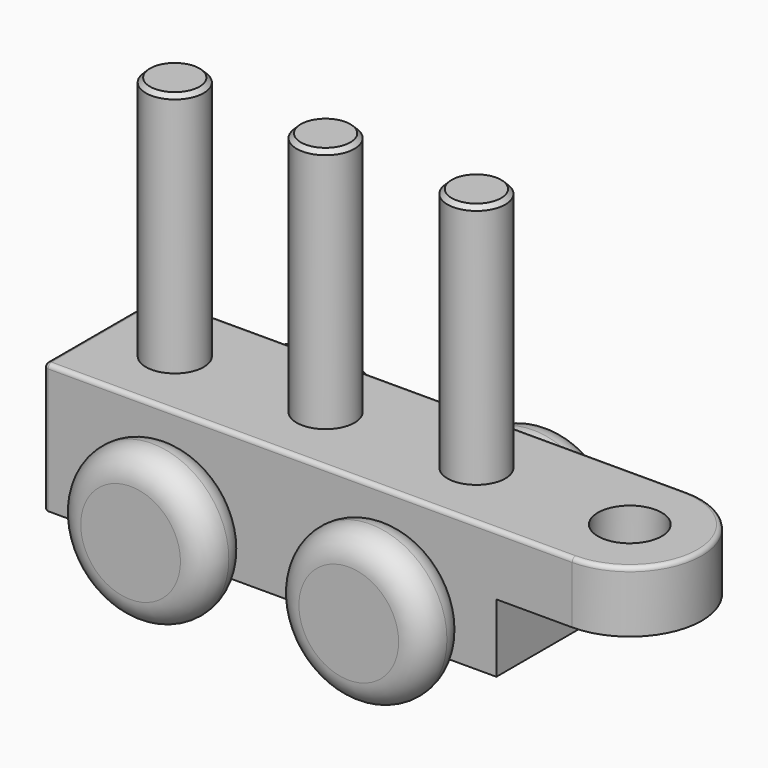
from build123d import *

# Parameters (mm, degrees)
F0_R           = 9.525
F1_DEPTH       = 38.608
F2_R           = 9.525
F3_DEPTH       = 20.32
F4_R           = 6.35
F5_DEPTH       = 42.926
F6_R           = 8.636
F7_DEPTH       = 73.152
F8_SIZE        = 1.27
F9_R           = 1.27
F10_R          = 6.35
F11_DEPTH      = 36.83
F12_R          = 22.86
F13_DEPTH      = 1.524
F13_DEPTH_BACK = 14.478
F12_R_2        = 6.35
F14_R          = 22.86
F14_R_2        = 6.35
F15_DEPTH      = 1.524
F15_DEPTH_BACK = 14.478
F16_R          = 8.00099
F16_2_R        = 8.00099
F16_3_R        = 8.00099
F16_4_R        = 8.00099


# Not quite as in the source:
# - a fillet or chamfer is up to 0.001 mm smaller than in the source, because OpenCascade refuses the exact size


with BuildPart() as f1:
    # F0 (on Top) → F1 (new body)
    with BuildSketch(Plane.XY):
        with BuildLine():
            Line((-21.463, 21.463), (-178.943, 21.463))
            Line((-178.943, 21.463), (-178.943, -21.463))
            Line((-178.943, -21.463), (-21.463, -21.463))
            ThreePointArc((-21.463, -21.463), (0, 0), (-21.463, 21.463))
        make_face()
        with Locations((-21.463, 0)):
            Circle(F0_R, mode=Mode.SUBTRACT)
    extrude(amount=F1_DEPTH)

    # F2 (on face) → F3 (cut)
    with BuildSketch(Plane(origin=(0, 0, 0), x_dir=(1, 0, 0), z_dir=(0, 0, -1))):
        with BuildLine():
            Line((-21.463, 21.463), (-44.069, 21.463))
            Line((-44.069, 21.463), (-44.069, -21.463))
            Line((-44.069, -21.463), (-21.463, -21.463))
            ThreePointArc((-21.463, -21.463), (0, 0), (-21.463, 21.463))
        make_face()
        with Locations((-21.463, 0)):
            Circle(F2_R, mode=Mode.SUBTRACT)
    extrude(amount=-F3_DEPTH, mode=Mode.SUBTRACT)

    # F4 (on face) → F5 (cut, through all)
    with BuildSketch(Plane.XZ.offset(21.463)):
        with Locations((-139.573, 10.922)):
            Circle(F4_R)
        with Locations((-74.549, 10.922)):
            Circle(F4_R)
    extrude(amount=-F5_DEPTH, mode=Mode.SUBTRACT)

    # F6 (on face) → F7 (join)
    with BuildSketch(Plane.XY.offset(38.608)):
        with Locations((-157.099, 0)):
            Circle(F6_R)
        with Locations((-112.141, 0)):
            Circle(F6_R)
        with Locations((-67.183, 0)):
            Circle(F6_R)
    extrude(amount=F7_DEPTH)

    # F8
    f8_edges = [f1.edges().sort_by_distance(p)[0] for p in [
        (-165.735, 0, 111.76),
        (-120.777, 0, 111.76),
        (-75.819, 0, 111.76),
    ]]
    chamfer(f8_edges, length=F8_SIZE)

    # F9
    f9_edges = [f1.edges().sort_by_distance(p)[0] for p in [
        (-100.203, 21.463, 38.608),
        (0, 0, 38.608),
        (-100.203, -21.463, 38.608),
        (-178.943, 0, 38.608),
        (-178.943, 21.463, 19.304),
        (-178.943, 0, 0),
        (-178.943, -21.463, 19.304),
    ]]
    fillet(f9_edges, radius=F9_R)


with BuildPart() as f11:
    # F10 (on Front) → F11 (new body, symmetric)
    with BuildSketch(Plane.XZ):
        with Locations((-139.573, 10.922)):
            Circle(F10_R)
    extrude(amount=F11_DEPTH, both=True)


with BuildPart() as f11b:
    # F10 (on Front) → F11, piece 2 (new body, symmetric)
    with BuildSketch(Plane.XZ):
        with Locations((-74.549, 10.922)):
            Circle(F10_R)
    extrude(amount=F11_DEPTH, both=True)


with BuildPart() as f13:
    # F12 (on face) → F13 (new body, two sides)
    with BuildSketch(Plane.XZ.offset(36.83)) as f13_sk:
        with Locations((-139.573, 10.922)):
            Circle(F12_R)
    extrude(amount=F13_DEPTH)
    extrude(f13_sk.sketch, amount=-F13_DEPTH_BACK)

    # F16 (radius 8.001 in the source; OpenCascade refuses exactly that, so slightly less here)
    f16_edges = [f13.edges().sort_by_distance(p)[0] for p in [
        (-162.433, -38.354, 10.922),
        (-162.433, -22.352, 10.922),
    ]]
    fillet(f16_edges, radius=F16_R)


with BuildPart() as f13b:
    # F12 (on face) → F13, piece 2 (new body, two sides)
    with BuildSketch(Plane.XZ.offset(36.83)) as f13_2_sk:
        with Locations((-74.549, 10.922)):
            Circle(F12_R)
        with Locations((-74.549, 10.922)):
            Circle(F12_R_2, mode=Mode.SUBTRACT)
        with Locations((-74.549, 10.922)):
            Circle(F12_R_2)
    extrude(amount=F13_DEPTH)
    extrude(f13_2_sk.sketch, amount=-F13_DEPTH_BACK)

    # F16#2 (radius 8.001 in the source; OpenCascade refuses exactly that, so slightly less here)
    f16_2_edges = [f13b.edges().sort_by_distance(p)[0] for p in [
        (-97.409, -38.354, 10.922),
        (-97.409, -22.352, 10.922),
    ]]
    fillet(f16_2_edges, radius=F16_2_R)


with BuildPart() as f15:
    # F14 (on face) → F15 (new body, two sides)
    with BuildSketch(Plane(origin=(0, 36.83, 0), x_dir=(-1, 0, 0), z_dir=(0, 1, 0))) as f15_sk:
        with Locations((139.573, 10.922)):
            Circle(F14_R)
        with Locations((139.573, 10.922)):
            Circle(F14_R_2, mode=Mode.SUBTRACT)
        with Locations((139.573, 10.922)):
            Circle(F14_R_2)
    extrude(amount=F15_DEPTH)
    extrude(f15_sk.sketch, amount=-F15_DEPTH_BACK)

    # F16#3 (radius 8.001 in the source; OpenCascade refuses exactly that, so slightly less here)
    f16_3_edges = [f15.edges().sort_by_distance(p)[0] for p in [
        (-116.713, 38.354, 10.922),
        (-116.713, 22.352, 10.922),
    ]]
    fillet(f16_3_edges, radius=F16_3_R)


with BuildPart() as f15b:
    # F14 (on face) → F15, piece 2 (new body, two sides)
    with BuildSketch(Plane(origin=(0, 36.83, 0), x_dir=(-1, 0, 0), z_dir=(0, 1, 0))) as f15_2_sk:
        with Locations((74.549, 10.922)):
            Circle(F14_R)
        with Locations((74.549, 10.922)):
            Circle(F14_R_2, mode=Mode.SUBTRACT)
        with Locations((74.549, 10.922)):
            Circle(F14_R_2)
    extrude(amount=F15_DEPTH)
    extrude(f15_2_sk.sketch, amount=-F15_DEPTH_BACK)

    # F16#4 (radius 8.001 in the source; OpenCascade refuses exactly that, so slightly less here)
    f16_4_edges = [f15b.edges().sort_by_distance(p)[0] for p in [
        (-51.689, 22.352, 10.922),
        (-51.689, 38.354, 10.922),
    ]]
    fillet(f16_4_edges, radius=F16_4_R)


solid = Compound([f1.part, f11.part, f11b.part, f13.part, f13b.part, f15.part, f15b.part])
